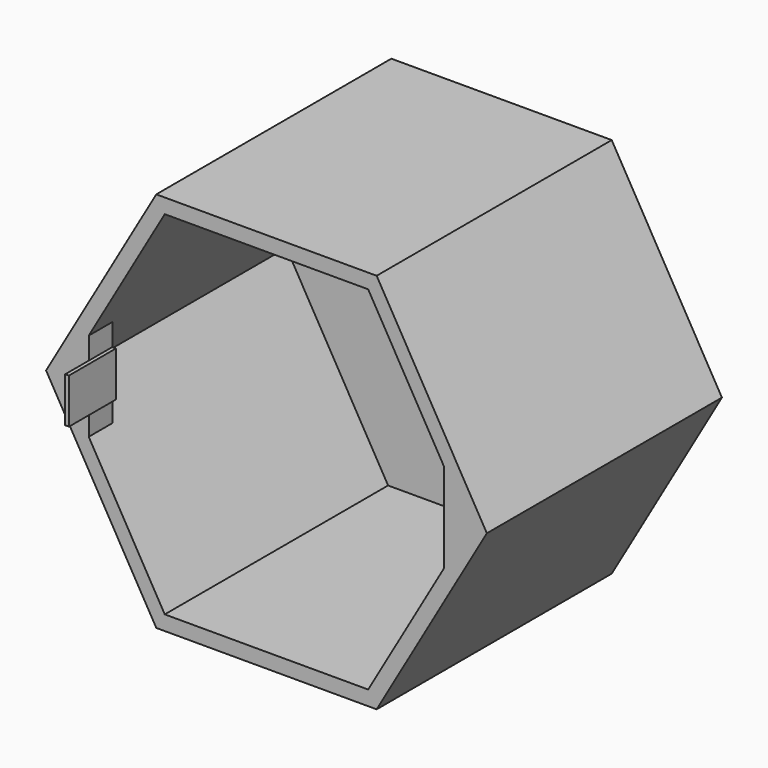
from build123d import *

# Parameters (mm, degrees)
F1_DEPTH  = 400
F2_T      = -20
F4_DEPTH  = 40
F5_W      = 40
F5_H      = 61.2435565298
F6_DEPTH  = 5
F7_W      = 5
F7_H      = 61.2435565298
F8_DEPTH  = 40
F9_W      = 20
F9_H      = 41.2435565298
F10_DEPTH = 20


with BuildPart() as f1:
    # F0 (on Front) → F1 (new body)
    with BuildSketch(Plane.XZ):
        Polygon((175.5110102277, 79.7711170535), (-124.4889897723, 79.7711170535), (-274.4889897723, -180.0365040818), (-124.4889897723, -439.8441252172), (175.5110102277, -439.8441252172), (325.5110102277, -180.0365040818), align=None)
    extrude(amount=F1_DEPTH)

    # F2
    f2_openings = [f1.faces().sort_by_distance(p)[0] for p in [
        (25.51101, -400, -180.036504),
    ]]
    offset(amount=F2_T, openings=f2_openings)

    # F3 (on face) → F4 (join)
    with BuildSketch(Plane.XZ.offset(400)):
        Polygon((175.5110102277, -439.8441252172), (325.5110102277, -180.0365040818), (175.5110102277, 79.7711170535), (-124.4889897723, 79.7711170535), (-274.4889897723, -180.0365040818), (-124.4889897723, -439.8441252172), align=None)
        Polygon((-216.3949790047, -240.6582823468), (-251.3949790047, -180.0365040818), (-216.3949790047, -119.4147258169), (-112.9419843885, 59.7711170535), (163.9640048439, 59.7711170535), (267.4169994601, -119.4147258169), (302.4169994601, -180.0365040818), (267.4169994601, -240.6582823468), (163.9640048439, -419.8441252172), (-112.9419843885, -419.8441252172), align=None, mode=Mode.SUBTRACT)
        Polygon((-216.3949790047, -119.4147258169), (-251.3949790047, -180.0365040818), (-216.3949790047, -240.6582823468), align=None)
        Polygon((302.4169994601, -180.0365040818), (267.4169994601, -119.4147258169), (267.4169994601, -240.6582823468), align=None)
    extrude(amount=-F4_DEPTH)

    # F5 (on face) → F6 (join)
    with BuildSketch(Plane.YZ.offset(-216.3949790047)):
        with Locations((-380, -180.0365040818)):
            Rectangle(F5_W, F5_H)
    extrude(amount=F6_DEPTH)

    # F7 (on face) → F8 (join)
    with BuildSketch(Plane.XZ.offset(400)):
        with Locations((-213.8949790047, -180.0365040818)):
            Rectangle(F7_W, F7_H)
    extrude(amount=F8_DEPTH)

    # F9 (on face) → F10 (cut)
    with BuildSketch(Plane(origin=(267.4169994601, 0, 0), x_dir=(0, -1, 0), z_dir=(-1, 0, 0))):
        with Locations((380.0858259201, -180.0365040818)):
            Rectangle(F9_W, F9_H)
    extrude(amount=-F10_DEPTH, mode=Mode.SUBTRACT)


solid = f1.part
